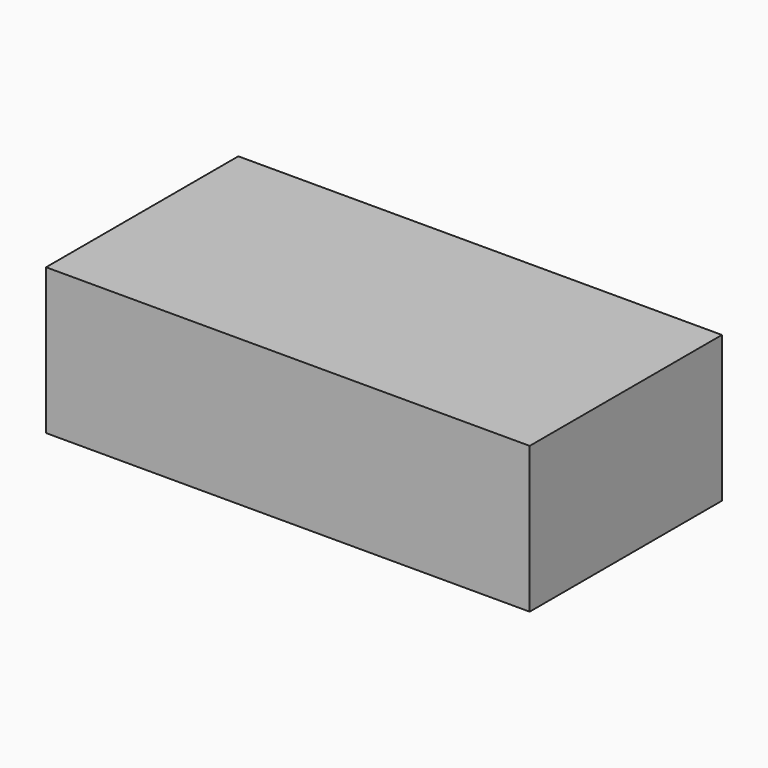
from build123d import *

# Parameters (mm, degrees)
F0_W     = 318
F0_H     = 158
F0_R     = 24
F1_DEPTH = 96


# Not quite as in the source:
# - a feature of the source that left no trace in its solid (it failed there, or was rolled back) is left out


with BuildPart() as f1:
    # F0 (on Top) → F1 (new body)
    with BuildSketch(Plane.XY):
        with Locations((159, 79)):
            Rectangle(F0_W, F0_H)
        with Locations((39, 39)):
            Circle(F0_R, mode=Mode.SUBTRACT)
        with Locations((119, 39)):
            Circle(F0_R, mode=Mode.SUBTRACT)
        with Locations((199, 39)):
            Circle(F0_R, mode=Mode.SUBTRACT)
        with Locations((279, 39)):
            Circle(F0_R, mode=Mode.SUBTRACT)
        with Locations((39, 119)):
            Circle(F0_R, mode=Mode.SUBTRACT)
        with Locations((119, 119)):
            Circle(F0_R, mode=Mode.SUBTRACT)
        with Locations((199, 119)):
            Circle(F0_R, mode=Mode.SUBTRACT)
        with Locations((279, 119)):
            Circle(F0_R, mode=Mode.SUBTRACT)
        with Locations((39, 39)):
            Circle(F0_R)
        with Locations((39, 119)):
            Circle(F0_R)
        with Locations((119, 119)):
            Circle(F0_R)
        with Locations((119, 39)):
            Circle(F0_R)
        with Locations((199, 119)):
            Circle(F0_R)
        with Locations((199, 39)):
            Circle(F0_R)
        with Locations((279, 39)):
            Circle(F0_R)
        with Locations((279, 119)):
            Circle(F0_R)
    extrude(amount=F1_DEPTH)


solid = f1.part
